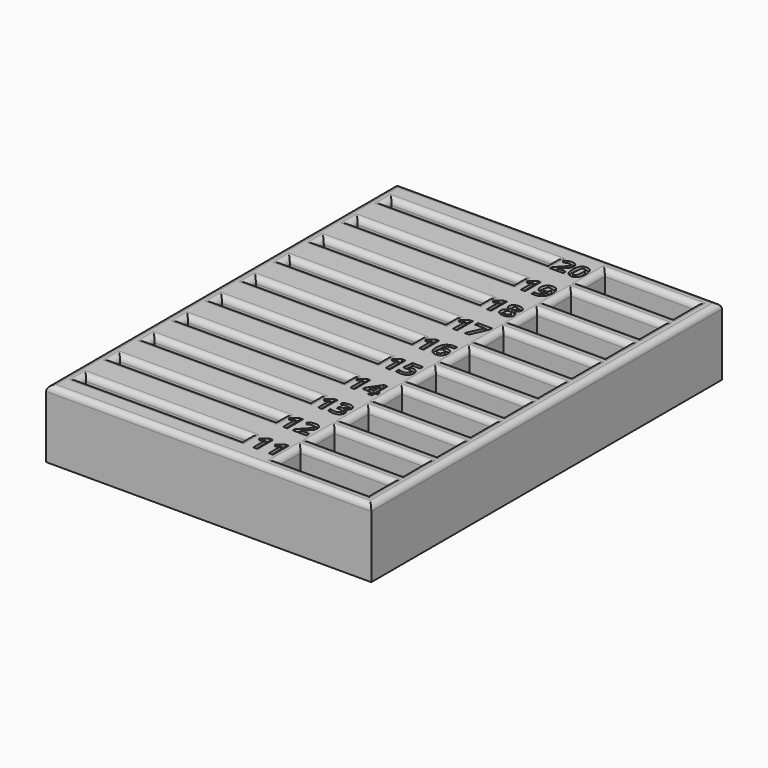
from build123d import *

# Parameters (mm, degrees)
F0_W           = 115
F0_H           = 155
F1_DEPTH       = 24
F2_W           = 32
F2_H           = 10
F2_W_2         = 57.5
F2_H_2         = 3
F3_DEPTH       = 23
F4_R           = 2
F2_TEXT_SIZE   = 9.7222222222
F2_TEXT_SIZE_2 = 9.4510783027
F2_TEXT_SIZE_3 = 9.312097811
F5_DEPTH       = 1


# Not quite as in the source:
# - a feature names something its author has since deleted; it is built from what else it names
# - Text() gives the source's letters only with a copy of the font that has no kerning and outlines rounded to 1/6400 em; it was checked with that copy


with BuildPart() as f1:
    # F0 (on Top) → F1 (new body)
    with BuildSketch(Plane.XY):
        with Locations((7.6503974199, 49.134781265)):
            Rectangle(F0_W, F0_H)
    extrude(amount=F1_DEPTH)

    # F2 (on face) → F3 (cut)
    with BuildSketch(Plane.XY.offset(24)):
        with Locations((44.1503974199, -18.365218735)):
            Rectangle(F2_W, F2_H)
        with Locations((-16.0996025801, -18.365218735)):
            Rectangle(F2_W_2, F2_H_2)
        with Locations((-16.11783728, -3.365218735)):
            Rectangle(F2_W_2, F2_H_2)
        with Locations((44.2294590175, -3.365218735)):
            Rectangle(F2_W, F2_H)
        with Locations((44.237555936, 11.634781265)):
            Rectangle(F2_W, F2_H)
        with Locations((44.0956111997, 26.634781265)):
            Rectangle(F2_W, F2_H)
        with Locations((43.9957920462, 41.634781265)):
            Rectangle(F2_W, F2_H)
        with Locations((43.9284516543, 56.634781265)):
            Rectangle(F2_W, F2_H)
        with Locations((43.9118291706, 71.634781265)):
            Rectangle(F2_W, F2_H)
        with Locations((43.8242364198, 86.634781265)):
            Rectangle(F2_W, F2_H)
        with Locations((43.7823194534, 101.634781265)):
            Rectangle(F2_W, F2_H)
        with Locations((43.7629665703, 116.634781265)):
            Rectangle(F2_W, F2_H)
        with Locations((-15.9132478945, 11.634781265)):
            Rectangle(F2_W_2, F2_H_2)
        with Locations((-16.0996025801, 26.634781265)):
            Rectangle(F2_W_2, F2_H_2)
        with Locations((-16.0996025801, 41.634781265)):
            Rectangle(F2_W_2, F2_H_2)
        with Locations((-16.0996025801, 56.634781265)):
            Rectangle(F2_W_2, F2_H_2)
        with Locations((-16.0996025801, 71.634781265)):
            Rectangle(F2_W_2, F2_H_2)
        with Locations((-16.0996025801, 86.634781265)):
            Rectangle(F2_W_2, F2_H_2)
        with Locations((-16.0996025801, 101.634781265)):
            Rectangle(F2_W_2, F2_H_2)
        with Locations((-16.0996025801, 116.634781265)):
            Rectangle(F2_W_2, F2_H_2)
    extrude(amount=-F3_DEPTH, mode=Mode.SUBTRACT)

    # F4
    f4_edges = [f1.edges().sort_by_distance(p)[0] for p in [
        (-16.099603, -19.865219, 24),
        (-16.099603, -16.865219, 24),
        (12.650397, -18.365219, 24),
        (-44.849603, -18.365219, 24),
        (44.150397, -13.365219, 24),
        (44.150397, -23.365219, 24),
        (28.150397, -18.365219, 24),
        (60.150397, -18.365219, 24),
        (-16.117837, -1.865219, 24),
        (-16.117837, -4.865219, 24),
        (-44.867837, -3.365219, 24),
        (12.632163, -3.365219, 24),
        (28.229459, -3.365219, 24),
        (44.229459, 1.634781, 24),
        (60.229459, -3.365219, 24),
        (44.229459, -8.365219, 24),
        (44.237556, 6.634781, 24),
        (28.237556, 11.634781, 24),
        (44.237556, 16.634781, 24),
        (60.237556, 11.634781, 24),
        (44.095611, 21.634781, 24),
        (60.095611, 26.634781, 24),
        (44.095611, 31.634781, 24),
        (28.095611, 26.634781, 24),
        (27.995792, 41.634781, 24),
        (43.995792, 46.634781, 24),
        (65.150397, 49.134781, 24),
        (7.650397, -28.365219, 24),
        (7.650397, 126.634781, 24),
        (-49.849603, 49.134781, 24),
        (12.836752, 11.634781, 24),
        (-15.913248, 13.134781, 24),
        (-44.663248, 11.634781, 24),
        (-15.913248, 10.134781, 24),
        (12.650397, 26.634781, 24),
        (-16.099603, 28.134781, 24),
        (-44.849603, 26.634781, 24),
        (-16.099603, 25.134781, 24),
        (-16.099603, 43.134781, 24),
        (-44.849603, 41.634781, 24),
        (-16.099603, 40.134781, 24),
        (12.650397, 41.634781, 24),
        (43.995792, 36.634781, 24),
        (59.995792, 41.634781, 24),
        (-16.099603, 58.134781, 24),
        (-44.849603, 56.634781, 24),
        (-16.099603, 55.134781, 24),
        (12.650397, 56.634781, 24),
        (-16.099603, 73.134781, 24),
        (-44.849603, 71.634781, 24),
        (-16.099603, 70.134781, 24),
        (12.650397, 71.634781, 24),
        (-16.099603, 88.134781, 24),
        (-44.849603, 86.634781, 24),
        (-16.099603, 85.134781, 24),
        (12.650397, 86.634781, 24),
        (-16.099603, 100.134781, 24),
        (12.650397, 101.634781, 24),
        (-16.099603, 103.134781, 24),
        (-44.849603, 101.634781, 24),
        (12.650397, 116.634781, 24),
        (-16.099603, 118.134781, 24),
        (-44.849603, 116.634781, 24),
        (-16.099603, 115.134781, 24),
        (59.928452, 56.634781, 24),
        (43.928452, 61.634781, 24),
        (27.928452, 56.634781, 24),
        (43.928452, 51.634781, 24),
        (43.911829, 66.634781, 24),
        (59.911829, 71.634781, 24),
        (43.911829, 76.634781, 24),
        (27.911829, 71.634781, 24),
        (59.824236, 86.634781, 24),
        (43.824236, 91.634781, 24),
        (27.824236, 86.634781, 24),
        (43.824236, 81.634781, 24),
        (59.782319, 101.634781, 24),
        (43.782319, 106.634781, 24),
        (27.782319, 101.634781, 24),
        (43.782319, 96.634781, 24),
        (43.762967, 121.634781, 24),
        (27.762967, 116.634781, 24),
        (43.762967, 111.634781, 24),
        (59.762967, 116.634781, 24),
    ]]
    fillet(f4_edges, radius=F4_R)

    # F2 (on face) → F5 (cut)
    with BuildSketch(Plane.XY.offset(24)):
        with Locations((14.3460617881, -7)):
            Text('12', F2_TEXT_SIZE, font='Open Sans', font_style=FontStyle.BOLD, text_align=(TextAlign.LEFT, TextAlign.BOTTOM))
        with Locations((14.7295473244, 8.0650821328)):
            Text('13', F2_TEXT_SIZE_2, font='Open Sans', font_style=FontStyle.BOLD, text_align=(TextAlign.LEFT, TextAlign.BOTTOM))
        with Locations((14.1895947742, 22.955543559)):
            Text('14', F2_TEXT_SIZE, font='Open Sans', font_style=FontStyle.BOLD, text_align=(TextAlign.LEFT, TextAlign.BOTTOM))
        with Locations((14.4736659548, 38.1669975966)):
            Text('15', F2_TEXT_SIZE, font='Open Sans', font_style=FontStyle.BOLD, text_align=(TextAlign.LEFT, TextAlign.BOTTOM))
        with Locations((14.3460617881, 53.2035712302)):
            Text('16', F2_TEXT_SIZE, font='Open Sans', font_style=FontStyle.BOLD, text_align=(TextAlign.LEFT, TextAlign.BOTTOM))
        with Locations((14.3460617881, 68.0930238366)):
            Text('17', F2_TEXT_SIZE, font='Open Sans', font_style=FontStyle.BOLD, text_align=(TextAlign.LEFT, TextAlign.BOTTOM))
        with Locations((14.3749246353, 83.0534171462)):
            Text('18', F2_TEXT_SIZE, font='Open Sans', font_style=FontStyle.BOLD, text_align=(TextAlign.LEFT, TextAlign.BOTTOM))
        with Locations((14.3749246353, 98.0639565885)):
            Text('19', F2_TEXT_SIZE, font='Open Sans', font_style=FontStyle.BOLD, text_align=(TextAlign.LEFT, TextAlign.BOTTOM))
        with Locations((14.8642051895, 113.0720302463)):
            Text('20', F2_TEXT_SIZE_3, font='Open Sans', font_style=FontStyle.BOLD, text_align=(TextAlign.LEFT, TextAlign.BOTTOM))
        with Locations((15.5704541492, -21.7896752805)):
            Text('11', F2_TEXT_SIZE, font='Open Sans', font_style=FontStyle.BOLD, text_align=(TextAlign.LEFT, TextAlign.BOTTOM))
    extrude(amount=-F5_DEPTH, mode=Mode.SUBTRACT)


solid = f1.part
